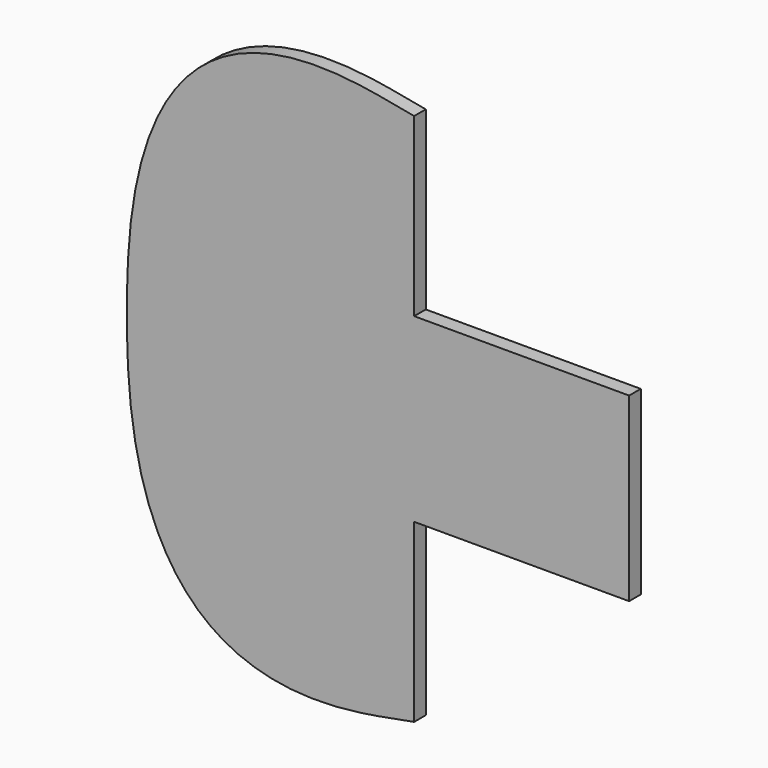
from build123d import *

# Parameters (mm, degrees)
F1_DEPTH    = 18
F2_T1_DEPTH = 18


# Not quite as in the source:
# - a fillet or chamfer that OpenCascade refuses, or shapes differently, is made with other operations: its cross-section is extruded or revolved along the edge and cut away or added


with BuildPart() as f1:
    # F0 (on Front) → F1 (new body)
    with BuildSketch(Plane.XZ):
        with BuildLine():
            Line((295, -217), (-326, -217))
            add(Edge.make_bspline(
                [(29, -547), (-32.3816202581, -555.0256740451), (-333.7546893929, -656.1166151476), (-326, -217)],
                knots=[0, 0, 0, 0, 484.6906229751, 484.6906229751, 484.6906229751, 484.6906229751], degree=3))
            Line((29, -547), (29, -329))
            Line((29, -329), (295, -329))
            Line((295, -329), (295, -217))
        make_face()
        with BuildLine():
            add(Edge.make_bspline(
                [(29, 113), (-32.3816202581, 121.0256740451), (-333.7546893929, 222.1166151476), (-326, -217)],
                knots=[0, 0, 0, 0, 484.6906229751, 484.6906229751, 484.6906229751, 484.6906229751], degree=3))
            Line((-326, -217), (295, -217))
            Line((295, -217), (295, -105))
            Line((295, -105), (29, -105))
            Line((29, -105), (29, 113))
        make_face()
    extrude(amount=F1_DEPTH)

    # F2: fillet of radius 100 on 1 edges, made by hand

    # F2_s2 → F2_t1 (join)
    with BuildSketch(Plane.XZ):
        with BuildLine():
            ThreePointArc((-326.0269192294, -218.5995282132), (-326.0141259586, -217), (-326.0269192294, -215.4004717868))
            ThreePointArc((-326.0269192294, -215.4004717868), (-326.0137919062, -216.2002414858), (-326, -217))
            ThreePointArc((-326, -217), (-326.0137919062, -217.7997585142), (-326.0269192294, -218.5995282132))
        make_face()
    extrude(amount=F2_T1_DEPTH)


solid = f1.part
